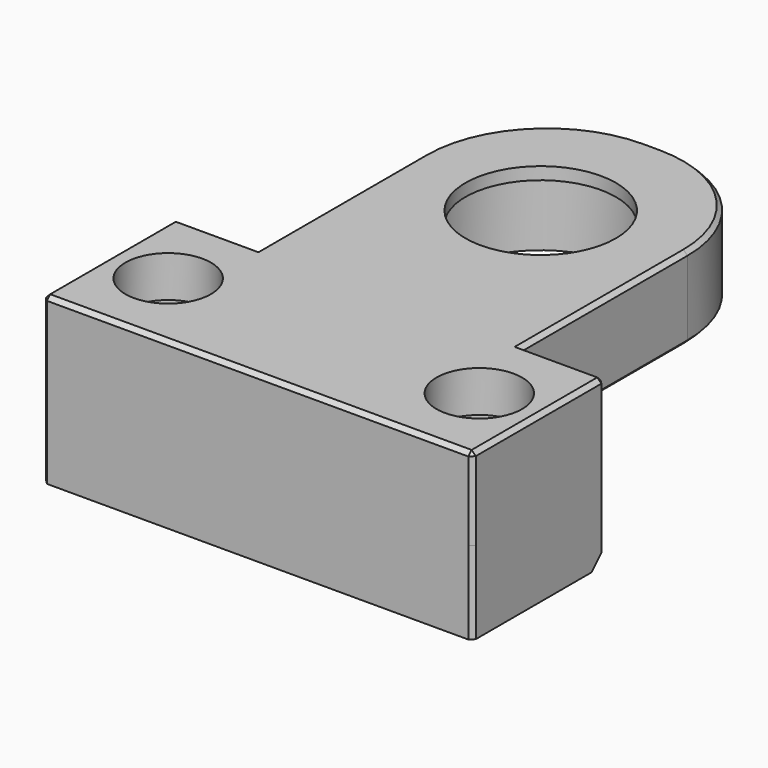
from build123d import *

# Parameters (mm, degrees)
F0_W      = 32
F0_H      = 40
F0_R      = 11.1
F0_R_2    = 5.175
F1_DEPTH  = 10
F0_R_3    = 2.675
F2_DEPTH  = 5
F3_DEPTH  = 5
F4_SIZE   = 0.5
F5_DEPTH  = 10
F6_DEPTH  = 10
F8_SIZE   = 2
F0_R_4    = 9.1
F9_DEPTH  = 10
F10_DEPTH = 8.5
F11_R     = 15
F12_SIZE  = 0.49999


# Not quite as in the source:
# - a fillet or chamfer is up to 0.001 mm smaller than in the source, because OpenCascade refuses the exact size
# - a feature of the source that left no trace in its solid (it failed there, or was rolled back) is left out


with BuildPart() as f1:
    # F0 (on Top) → F1 (new body)
    with BuildSketch(Plane.XY):
        with Locations((-1.076085493, 10.825)):
            Rectangle(F0_W, F0_H)
        with Locations((-1.076085493, 13.645)):
            Circle(F0_R, mode=Mode.SUBTRACT)
        Polygon((14.923914507, -9.175), (-17.076085493, -9.175), (-27.076085493, -9.175), (-27.076085493, -29.175), (-17.076085493, -29.175), (14.923914507, -29.175), (24.923914507, -29.175), (24.923914507, -9.175), align=None)
        with Locations((-19.901085493, -19.175)):
            Circle(F0_R_2, mode=Mode.SUBTRACT)
        with Locations((17.748914507, -19.175)):
            Circle(F0_R_2, mode=Mode.SUBTRACT)
    extrude(amount=F1_DEPTH)

    # F0 (on Top) → F2 (join)
    with BuildSketch(Plane.XY):
        with Locations((-19.901085493, -19.175)):
            Circle(F0_R_2)
        with Locations((-19.901085493, -19.175)):
            Circle(F0_R_3, mode=Mode.SUBTRACT)
    extrude(amount=F2_DEPTH)

    # F0 (on Top) → F3 (join)
    with BuildSketch(Plane.XY):
        with Locations((17.748914507, -19.175)):
            Circle(F0_R_2)
        with Locations((17.748914507, -19.175)):
            Circle(F0_R_3, mode=Mode.SUBTRACT)
    extrude(amount=F3_DEPTH)

    # F4
    f4_edges = [f1.edges().sort_by_distance(p)[0] for p in [
        (-27.076085, -19.175, 10),
        (-22.076085, -9.175, 10),
        (19.923915, -9.175, 10),
        (24.923915, -19.175, 10),
        (24.923915, -9.175, 5),
        (-27.076085, -9.175, 5),
        (-27.076085, -29.175, 5),
        (24.923915, -29.175, 5),
        (-1.076085, -29.175, 10),
        (-17.076085, 10.825, 10),
        (14.923915, 10.825, 10),
    ]]
    chamfer(f4_edges, length=F4_SIZE)

    # F0 (on Top) → F5 (join)
    with BuildSketch(Plane.XY):
        Polygon((14.923914507, -9.175), (-17.076085493, -9.175), (-27.076085493, -9.175), (-27.076085493, -29.175), (-17.076085493, -29.175), (14.923914507, -29.175), (24.923914507, -29.175), (24.923914507, -9.175), align=None)
        with Locations((-19.901085493, -19.175)):
            Circle(F0_R_2, mode=Mode.SUBTRACT)
        with Locations((17.748914507, -19.175)):
            Circle(F0_R_2, mode=Mode.SUBTRACT)
    extrude(amount=-F5_DEPTH)

    # F0 (on Top) → F6 (join)
    with BuildSketch(Plane.XY):
        with Locations((17.748914507, -19.175)):
            Circle(F0_R_2)
        with Locations((17.748914507, -19.175)):
            Circle(F0_R_3, mode=Mode.SUBTRACT)
        with Locations((-19.901085493, -19.175)):
            Circle(F0_R_2)
        with Locations((-19.901085493, -19.175)):
            Circle(F0_R_3, mode=Mode.SUBTRACT)
    extrude(amount=-F6_DEPTH)

    # F8
    f8_edges = [f1.edges().sort_by_distance(p)[0] for p in [
        (-1.076085, -9.175, -10),
    ]]
    chamfer(f8_edges, length=F8_SIZE)

    # F0 (on Top) → F9 (join)
    with BuildSketch(Plane.XY):
        with Locations((-1.076085493, 13.645)):
            Circle(F0_R)
        with Locations((-1.076085493, 13.645)):
            Circle(F0_R_4, mode=Mode.SUBTRACT)
    extrude(amount=F9_DEPTH)

    # F0 (on Top) → F10 (cut)
    with BuildSketch(Plane.XY):
        with Locations((-1.076085493, 13.645)):
            Circle(F0_R)
        with Locations((-1.076085493, 13.645)):
            Circle(F0_R_4, mode=Mode.SUBTRACT)
    extrude(amount=F10_DEPTH, mode=Mode.SUBTRACT)

    # F11
    f11_edges = [f1.edges().sort_by_distance(p)[0] for p in [
        (14.923915, 30.825, 4.75),
        (-17.076085, 30.825, 4.75),
    ]]
    fillet(f11_edges, radius=F11_R)

    # F12 (size 0.5 in the source; OpenCascade refuses exactly that, so slightly less here)
    f12_edges = [f1.edges().sort_by_distance(p)[0] for p in [
        (10.530516, 26.431602, 0),
        (-11.224621, 27.712148, 10),
        (9.07245, 27.712148, 10),
        (-1.076085, 30.825, 10),
        (-1.076085, 30.825, 0),
        (-12.682687, 26.431602, 0),
        (-17.076085, 3.325, 0),
        (-27.076085, -9.175, -4),
        (24.923915, -9.175, -4),
        (14.923915, 3.325, 0),
        (-27.076085, -29.175, -5),
        (24.923915, -29.175, -5),
    ]]
    chamfer(f12_edges, length=F12_SIZE)


solid = f1.part
